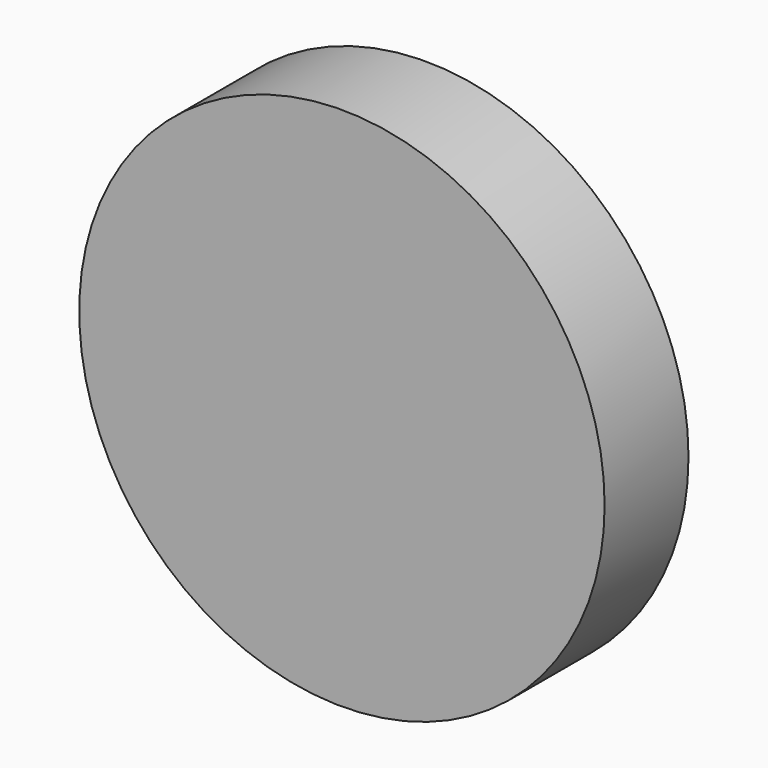
from build123d import *

# Parameters (mm, degrees)
F0_R     = 63.6332649279
F1_DEPTH = 25.4


# Not quite as in the source:
# - the program builds the solid bodies; features that only make, move or delete a surface that nothing else refers to are left out


with BuildPart() as f1:
    # F0 (on Front) → F1 (new body)
    with BuildSketch(Plane.XZ):
        Circle(F0_R)
    extrude(amount=F1_DEPTH)


solid = f1.part
